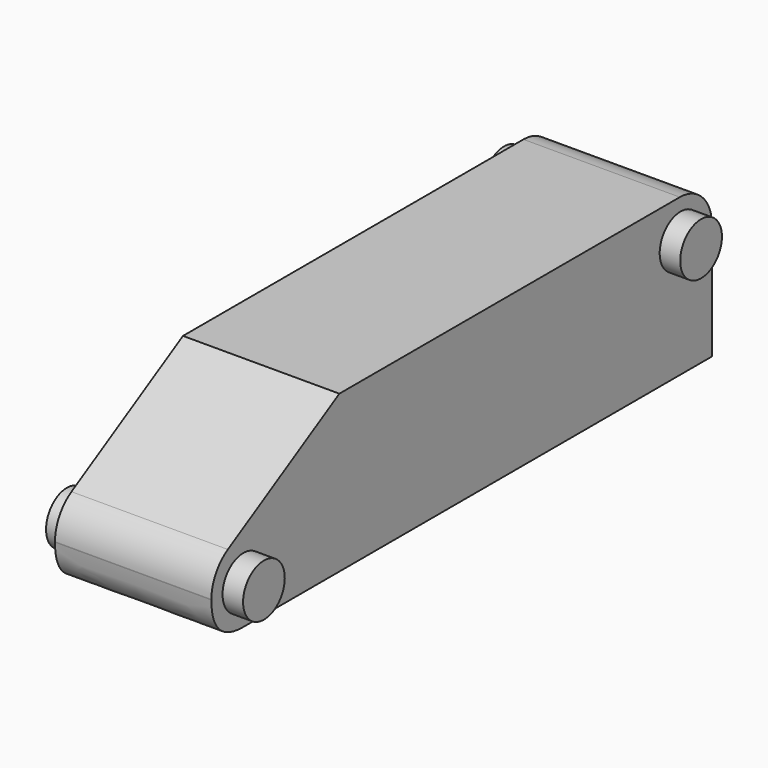
from build123d import *

# Parameters (mm, degrees)
F0_W           = 304.8
F0_H           = 76.3
F1_DEPTH       = 3
F2_DEPTH       = 76.2
F3_T1_DEPTH    = 173.7
F4_R           = 19.5
F5_T1_DEPTH    = 479.4867573526
F6_R           = 20.0387150069
F8_R           = 12.7
F9_DEPTH       = 10
F9_DEPTH_BACK  = 86
F10_R          = 12.7
F11_DEPTH      = 10
F11_DEPTH_BACK = 86


# Not quite as in the source:
# - a fillet or chamfer that OpenCascade refuses, or shapes differently, is made with other operations: its cross-section is extruded or revolved along the edge and cut away or added


with BuildPart() as f1:
    # F0 (on Right) → F1 (new body)
    with BuildSketch(Plane.YZ):
        with Locations((152.4, 38.15)):
            Rectangle(F0_W, F0_H)
    extrude(amount=F1_DEPTH)

    # F0 (on Right) → F2 (join)
    with BuildSketch(Plane.YZ):
        with Locations((152.4, 38.15)):
            Rectangle(F0_W, F0_H)
    extrude(amount=F2_DEPTH)

    # F3: fillet of radius 19.5 on 1 edges, made by hand

    # F3_s2 → F3_t1 (cut)
    with BuildSketch(Plane.YZ.offset(-48.75)):
        with BuildLine():
            add(Edge.make_bspline(
                [(0, 19.5), (0, 0), (19.5, 0)],
                knots=[0, 0, 0, 1, 1, 1], degree=2, weights=[1, 1, 1]))
            Line((19.5, 0), (0, 0))
            Line((0, 0), (0, 19.5))
        make_face()
    extrude(amount=F3_T1_DEPTH, mode=Mode.SUBTRACT)

    # F4
    f4_edges = [f1.edges().sort_by_distance(p)[0] for p in [
        (38.1, 304.8, 76.3),
    ]]
    fillet(f4_edges, radius=F4_R)

    # F5: chamfer of 45 x 77.9422863406 on 1 edges, made by hand

    # F5_s2 → F5_t1 (cut)
    with BuildSketch(Plane.YZ.offset(-201.6433786763)):
        Polygon((77.9422863406, 76.3), (0, 31.3), (0, 76.3), align=None)
    extrude(amount=F5_T1_DEPTH, mode=Mode.SUBTRACT)

    # F6
    f6_edges = [f1.edges().sort_by_distance(p)[0] for p in [
        (38.1, 0, 31.3),
    ]]
    fillet(f6_edges, radius=F6_R)

    # F8 (on offset) → F9 (join, two sides)
    with BuildSketch(Plane.YZ.offset(76.2)) as f9_sk:
        with Locations((19.4881175538, 19.05)):
            Circle(F8_R)
    extrude(amount=F9_DEPTH)
    extrude(f9_sk.sketch, amount=-F9_DEPTH_BACK)

    # F10 (on offset) → F11 (join, two sides)
    with BuildSketch(Plane.YZ.offset(76.2)) as f11_sk:
        with Locations((285.75, 57.25)):
            Circle(F10_R)
    extrude(amount=F11_DEPTH)
    extrude(f11_sk.sketch, amount=-F11_DEPTH_BACK)


solid = f1.part
